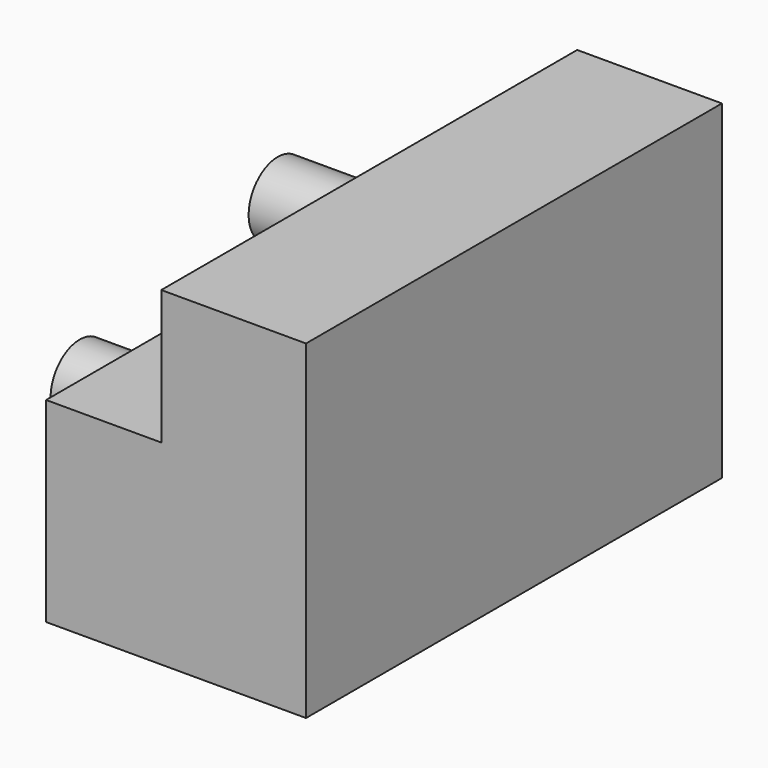
from build123d import *

# Parameters (mm, degrees)
F1_DEPTH = 50
F2_R     = 3.5
F3_DEPTH = 10
F4_R     = 3.5
F5_DEPTH = 10
F6_R     = 3.5
F7_DEPTH = 10


# Not quite as in the source:
# - a feature names something its author has since deleted; it is built from what else it names


with BuildPart() as f1:
    # F0 (on Front) → F1 (new body)
    with BuildSketch(Plane.XZ):
        Polygon((0, -6.7148432136), (25, -6.7148432136), (25, 25), (11.0791092739, 25), (11.0791092739, 12.0865814388), (0, 12.0865814388), align=None)
    extrude(amount=F1_DEPTH)

    # F2 (on face) → F3 (join)
    with BuildSketch(Plane(origin=(0, 0, 0), x_dir=(0, -1, 0), z_dir=(-1, 0, 0))):
        with Locations((13.8432676521, 3.730392782)):
            Circle(F2_R)
        with Locations((33.459926671, 3.730392782)):
            Circle(F2_R)
    extrude(amount=F3_DEPTH)

    # F4 (on face) → F5 (cut)
    with BuildSketch(Plane(origin=(0, 0, -6.7148432136), x_dir=(1, 0, 0), z_dir=(0, 0, -1))):
        with Locations((12.6557382198, 36.55)):
            Circle(F4_R)
        with Locations((13.0857451583, 13.4541578871)):
            Circle(F4_R)
    extrude(amount=-F5_DEPTH, mode=Mode.SUBTRACT)

    # F6 (on face) → F7 (join)
    with BuildSketch(Plane(origin=(11.0791092739, 0, 0), x_dir=(0, -1, 0), z_dir=(-1, 0, 0))):
        with Locations((23.5, 18.7478940934)):
            Circle(F6_R)
    extrude(amount=F7_DEPTH)


solid = f1.part
